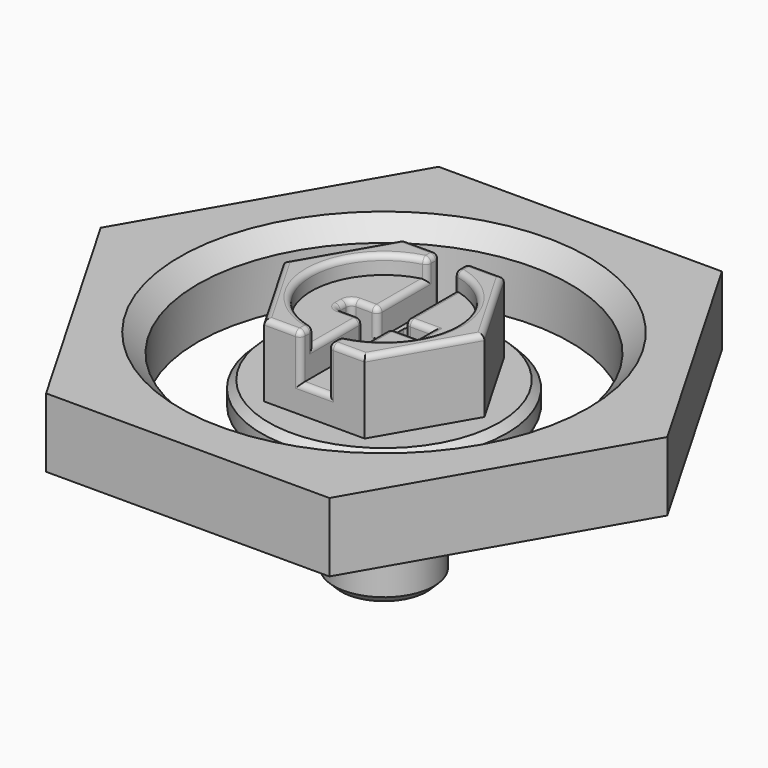
from build123d import *

# Parameters (mm, degrees)
F0_R          = 10.25
F1_DEPTH      = 3.8
F2_SIZE       = 1
F3_R          = 2.75
F4_DEPTH      = 8
F3_R_2        = 6.75
F5_DEPTH      = 1.5
F7_DEPTH      = 4
F8_R          = 4
F9_DEPTH      = 1
F11_DEPTH     = 2.5
F12_W         = 1.75
F12_H         = 1
F12_W_2       = 1
F12_H_2       = 1.75
F12_W_3       = 1.5
F12_W_4       = 0.25
F13_DEPTH     = 2.5
F14_R         = 0.3
F15_T1_DEPTH  = 1.2
F15_S5_W      = 0.3
F15_S5_H      = 0.3
F15_T6_DEPTH  = 0.3
F15_S11_W     = 0.3
F15_S11_H     = 0.3
F15_T12_DEPTH = 0.3
F15_S17_W     = 0.3
F15_S17_H     = 0.3
F15_T18_DEPTH = 0.3
F15_S23_W     = 0.3
F15_S23_H     = 0.3
F15_T24_DEPTH = 0.3
F16_R         = 0.3
F17_SIZE      = 0.4


# Not quite as in the source:
# - a fillet or chamfer that OpenCascade refuses, or shapes differently, is made with other operations: its cross-section is extruded or revolved along the edge and cut away or added


with BuildPart() as f1:
    # F0 (on Top) → F1 (new body)
    with BuildSketch(Plane.XY):
        Polygon((7.794, 13.4996039942), (-7.794, 13.4996039942), (-15.588, 0), (-7.794, -13.4996039942), (7.794, -13.4996039942), (15.588, 0), align=None)
        Circle(F0_R, mode=Mode.SUBTRACT)
    extrude(amount=F1_DEPTH)

    # F2
    f2_edges = [f1.edges().sort_by_distance(p)[0] for p in [
        (-10.25, 0, 3.8),
    ]]
    chamfer(f2_edges, length=F2_SIZE)


with BuildPart() as f4:
    # F3 (on Top) → F4 (new body)
    with BuildSketch(Plane.XY):
        Circle(F3_R)
    extrude(amount=-F4_DEPTH)

    # F3 (on Top) → F5 (join)
    with BuildSketch(Plane.XY):
        Circle(F3_R_2)
        Circle(F3_R, mode=Mode.SUBTRACT)
        Circle(F3_R)
    extrude(amount=F5_DEPTH)

    # F6 (on face) → F7 (join)
    with BuildSketch(Plane.XY.offset(1.5)):
        Polygon((2.7625, 4.7847903559), (-2.7625, 4.7847903559), (-5.525, 0), (-2.7625, -4.7847903559), (2.7625, -4.7847903559), (5.525, 0), align=None)
    extrude(amount=F7_DEPTH)

    # F8 (on face) → F9 (cut)
    with BuildSketch(Plane.XY.offset(5.5)):
        Circle(F8_R)
    extrude(amount=-F9_DEPTH, mode=Mode.SUBTRACT)

    # F10 (on face) → F11 (cut)
    with BuildSketch(Plane.XY.offset(5.5)):
        with BuildLine():
            Line((0.75, 4.7847903559), (-0.75, 4.7847903559))
            Line((-0.75, 4.7847903559), (-0.75, 3.9290584114))
            ThreePointArc((-0.75, 3.9290584114), (0, 4), (0.75, 3.9290584114))
            Line((0.75, 3.9290584114), (0.75, 4.7847903559))
        make_face()
        with BuildLine():
            ThreePointArc((0.75, 3.9290584114), (0, 4), (-0.75, 3.9290584114))
            Line((-0.75, 3.9290584114), (-0.75, -3.9290584114))
            ThreePointArc((-0.75, -3.9290584114), (0, -4), (0.75, -3.9290584114))
            Line((0.75, -3.9290584114), (0.75, 3.9290584114))
        make_face()
        with BuildLine():
            ThreePointArc((0.75, -3.9290584114), (0, -4), (-0.75, -3.9290584114))
            Line((-0.75, -3.9290584114), (-0.75, -4.7847903559))
            Line((-0.75, -4.7847903559), (0.75, -4.7847903559))
            Line((0.75, -4.7847903559), (0.75, -3.9290584114))
        make_face()
    extrude(amount=-F11_DEPTH, mode=Mode.SUBTRACT)

    # F12 (on face) → F13 (cut)
    with BuildSketch(Plane.XY.offset(4.5)):
        with Locations((1.375, 0)):
            Rectangle(F12_W, F12_H)
        Rectangle(F12_W_2, F12_H)
        with Locations((0, 1.375)):
            Rectangle(F12_W_2, F12_H_2)
        with Locations((0, -1.375)):
            Rectangle(F12_W_2, F12_H_2)
        with Locations((-1.5, 0)):
            Rectangle(F12_W_3, F12_H)
        with Locations((-0.625, 0)):
            Rectangle(F12_W_4, F12_H)
    extrude(amount=-F13_DEPTH, mode=Mode.SUBTRACT)

    # F14
    f14_edges = [f4.edges().sort_by_distance(p)[0] for p in [
        (-0.75, 4.356924, 5.5),
        (-4, 0, 5.5),
        (-0.75, -4.356924, 5.5),
        (-1.75625, -4.78479, 5.5),
        (-4.14375, -2.392395, 5.5),
        (-4.14375, 2.392395, 5.5),
        (-1.75625, 4.78479, 5.5),
        (4.14375, 2.392395, 5.5),
        (1.75625, 4.78479, 5.5),
        (0.75, 4.356924, 5.5),
        (4, 0, 5.5),
        (0.75, -4.356924, 5.5),
        (1.75625, -4.78479, 5.5),
        (4.14375, -2.392395, 5.5),
        (-0.75, -4.78479, 4.25),
        (0, -4.78479, 3),
        (0.75, -4.78479, 4.25),
        (-0.75, 4.78479, 4.25),
        (0, 4.78479, 3),
        (0.75, 4.78479, 4.25),
        (0.75, -2.214529, 4.5),
        (0.75, 2.214529, 4.5),
        (0.75, 3.929058, 5),
        (0.75, -3.929058, 5),
        (1.5, 0.5, 4.5),
        (2.25, 0, 4.5),
        (1.5, -0.5, 4.5),
        (-0.75, -3.929058, 5),
        (-0.75, 3.929058, 5),
        (-0.75, -2.214529, 4.5),
        (-1.5, -0.5, 4.5),
        (-1.5, 0.5, 4.5),
        (-2.25, 0, 4.5),
        (-0.75, 2.214529, 4.5),
        (-0.5, 2.25, 2.5),
        (0.5, 2.25, 2.5),
        (0.5, -2.25, 2.5),
        (-0.5, -2.25, 2.5),
        (-2.25, -0.5, 3.25),
        (-2.25, 0.5, 3.25),
    ]]
    fillet(f14_edges, radius=F14_R)

    # F15: fillet of radius 0.3 on 4 edges, made by hand

    # F15_s2 → F15_t1 (cut)
    with BuildSketch(Plane.XY.offset(3)):
        with BuildLine():
            ThreePointArc((0.75, -0.8), (0.8378679656, -0.5878679656), (1.05, -0.5))
            Line((1.05, -0.5), (0.75, -0.5))
            Line((0.75, -0.5), (0.75, -0.8))
        make_face()
        with BuildLine():
            ThreePointArc((0.75, 0.8), (0.8378679656, 0.5878679656), (1.05, 0.5))
            Line((1.05, 0.5), (0.75, 0.5))
            Line((0.75, 0.5), (0.75, 0.8))
        make_face()
        with BuildLine():
            ThreePointArc((-0.75, 0.8), (-0.8378679656, 0.5878679656), (-1.05, 0.5))
            Line((-1.05, 0.5), (-0.75, 0.5))
            Line((-0.75, 0.5), (-0.75, 0.8))
        make_face()
        with BuildLine():
            ThreePointArc((-0.75, -0.8), (-0.8378679656, -0.5878679656), (-1.05, -0.5))
            Line((-1.05, -0.5), (-0.75, -0.5))
            Line((-0.75, -0.5), (-0.75, -0.8))
        make_face()
    extrude(amount=F15_T1_DEPTH, mode=Mode.SUBTRACT)


with BuildPart() as f15_tool4:
    # F15_s5 → F15_t6 (new body)
    with BuildSketch(Plane.YZ.offset(-1.05)):
        with Locations((-0.65, 4.35)):
            Rectangle(F15_S5_W, F15_S5_H)
    extrude(amount=F15_T6_DEPTH)

    # F15_s7 → F15_t8 (revolve, cut)
    with BuildSketch(Plane(origin=(-1.05, -0.8, 4.2), x_dir=(0, -0.7071067812, -0.7071067812), z_dir=(0, -0.7071067812, 0.7071067812))):
        with BuildLine():
            ThreePointArc((0, -0.3), (0.3, 0), (0, 0.3))
            Line((0, 0.3), (0, -0.3))
        make_face()
    revolve(axis=Axis((-1.05, -0.8, 4.2), (1, 0, 0)), mode=Mode.SUBTRACT)


with BuildPart() as f4_1:
    add(f4.part)

    # F15_t3: cut F15_tool4
    add(f15_tool4.part, mode=Mode.SUBTRACT)


with BuildPart() as f15_tool10:
    # F15_s11 → F15_t12 (new body)
    with BuildSketch(Plane.YZ.offset(-1.05)):
        with Locations((0.65, 4.35)):
            Rectangle(F15_S11_W, F15_S11_H)
    extrude(amount=F15_T12_DEPTH)

    # F15_s13 → F15_t14 (revolve, cut)
    with BuildSketch(Plane(origin=(-1.05, 0.8, 4.2), x_dir=(0, 0.7071067812, -0.7071067812), z_dir=(0, -0.7071067812, -0.7071067812))):
        with BuildLine():
            ThreePointArc((0, -0.3), (0.3, 0), (0, 0.3))
            Line((0, 0.3), (0, -0.3))
        make_face()
    revolve(axis=Axis((-1.05, 0.8, 4.2), (1, 0, 0)), mode=Mode.SUBTRACT)


with BuildPart() as f4_2:
    add(f4_1.part)

    # F15_t9: cut F15_tool10
    add(f15_tool10.part, mode=Mode.SUBTRACT)


with BuildPart() as f15_tool16:
    # F15_s17 → F15_t18 (new body)
    with BuildSketch(Plane.YZ.offset(1.05)):
        with Locations((0.65, 4.35)):
            Rectangle(F15_S17_W, F15_S17_H)
    extrude(amount=-F15_T18_DEPTH)

    # F15_s19 → F15_t20 (revolve, cut)
    with BuildSketch(Plane(origin=(1.05, 0.8, 4.2), x_dir=(0, 0.7071067812, -0.7071067812), z_dir=(0, 0.7071067812, 0.7071067812))):
        with BuildLine():
            ThreePointArc((0, -0.3), (0.3, 0), (0, 0.3))
            Line((0, 0.3), (0, -0.3))
        make_face()
    revolve(axis=Axis((1.05, 0.8, 4.2), (-1, 0, 0)), mode=Mode.SUBTRACT)


with BuildPart() as f4_3:
    add(f4_2.part)

    # F15_t15: cut F15_tool16
    add(f15_tool16.part, mode=Mode.SUBTRACT)


with BuildPart() as f15_tool22:
    # F15_s23 → F15_t24 (new body)
    with BuildSketch(Plane.YZ.offset(1.05)):
        with Locations((-0.65, 4.35)):
            Rectangle(F15_S23_W, F15_S23_H)
    extrude(amount=-F15_T24_DEPTH)

    # F15_s25 → F15_t26 (revolve, cut)
    with BuildSketch(Plane(origin=(1.05, -0.8, 4.2), x_dir=(0, -0.7071067812, -0.7071067812), z_dir=(0, 0.7071067812, -0.7071067812))):
        with BuildLine():
            ThreePointArc((0, -0.3), (0.3, 0), (0, 0.3))
            Line((0, 0.3), (0, -0.3))
        make_face()
    revolve(axis=Axis((1.05, -0.8, 4.2), (-1, 0, 0)), mode=Mode.SUBTRACT)


with BuildPart() as f4_4:
    add(f4_3.part)

    # F15_t21: cut F15_tool22
    add(f15_tool22.part, mode=Mode.SUBTRACT)

    # F16
    f16_edges = [f4_4.edges().sort_by_distance(p)[0] for p in [
        (0.5, 0.5, 2.5),
        (-0.5, 0.5, 2.5),
        (-0.5, -0.5, 2.5),
        (0.5, -0.5, 2.5),
        (-6.75, 0, 0),
    ]]
    fillet(f16_edges, radius=F16_R)

    # F17
    f17_edges = [f4_4.edges().sort_by_distance(p)[0] for p in [
        (-6.75, 0, 1.5),
        (-2.75, 0, -8),
    ]]
    chamfer(f17_edges, length=F17_SIZE)


solid = Compound([f1.part, f4_4.part])
